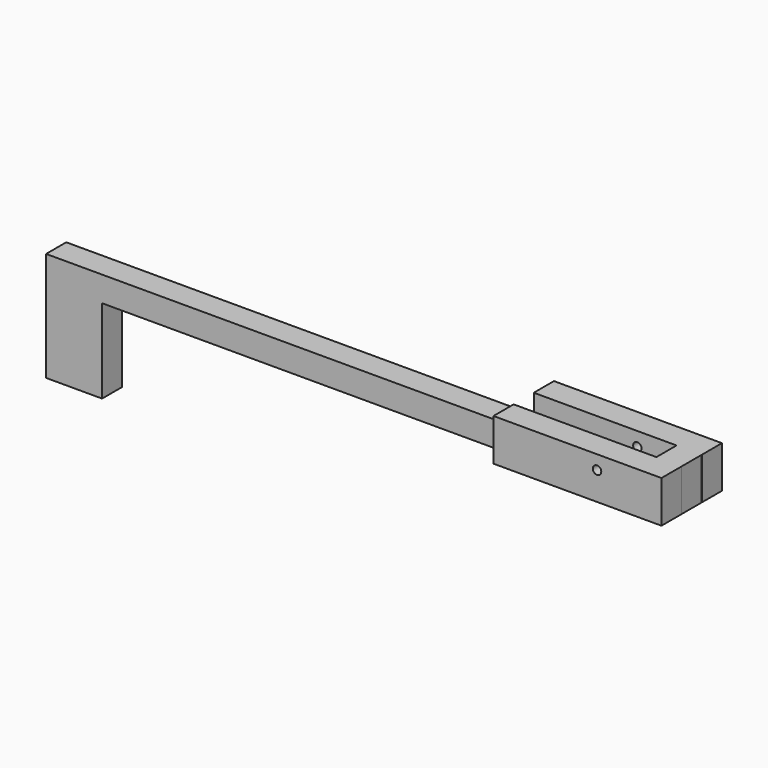
from build123d import *

# Parameters (mm, degrees)
F0_W     = 20
F0_H     = 30
F1_DEPTH = 4.5
F0_W_2   = 9
F0_H_2   = 15
F3_W     = 60
F3_H     = 15
F3_R     = 1.5
F4_DEPTH = 9


with BuildPart() as f1:
    # F0 (on Front) → F1 (new body, symmetric)
    with BuildSketch(Plane.XZ):
        Polygon((177, 9), (0, 9), (0, 0), (20, 0), (177, 0), align=None)
        with Locations((10, -15)):
            Rectangle(F0_W, F0_H)
    extrude(amount=F1_DEPTH, both=True)



with BuildPart() as f1b:
    # F0 (on Front) → F1, piece 2 (new body, symmetric)
    with BuildSketch(Plane.XZ):
        with Locations((222.4899989998, 8.5)):
            Rectangle(F0_W_2, F0_H_2)
    extrude(amount=F1_DEPTH, both=True)


with BuildPart() as f1_1:
    add(f1.part)

    add(f1b.part)  # F4 merges F1b
    # F3 (on offset) → F4 (join)
    with BuildSketch(Plane.XZ.offset(-4.5)):
        with Locations((197, 8.5)):
            Rectangle(F3_W, F3_H)
        with Locations((204, 11)):
            Circle(F3_R, mode=Mode.SUBTRACT)
    extrude(amount=-F4_DEPTH)

    # F5: F1 across plane


with BuildPart() as f1_2:
    add(f1_1.part)
    add(f1_1.part.mirror(Plane.XZ))


solid = f1_2.part
